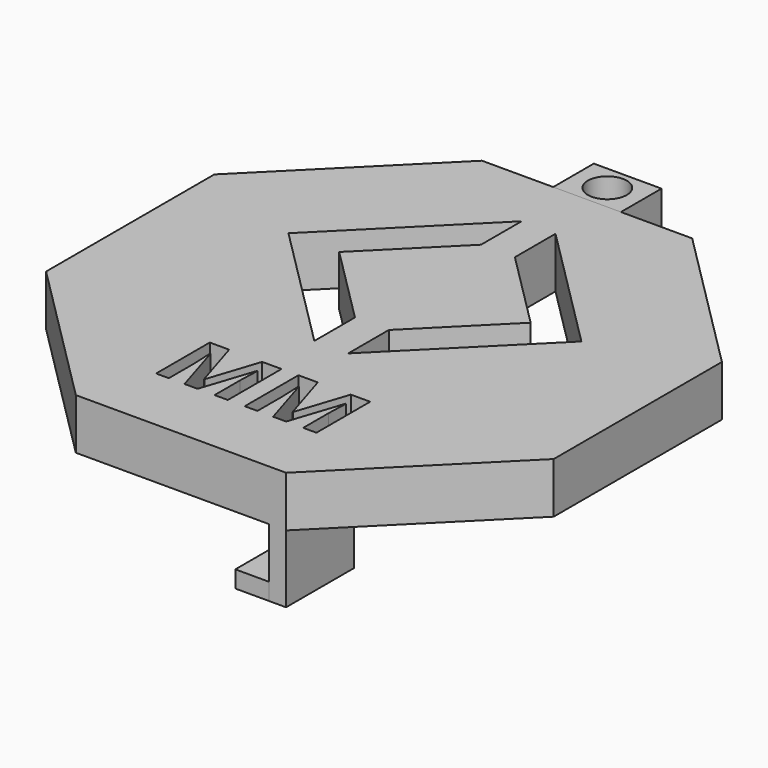
from build123d import *

# Parameters (mm, degrees)
F1_DEPTH     = 3
F2_TEXT_SIZE = 5.5555555556
F3_DEPTH     = 3.001
F4_W         = 1
F4_H         = 5
F5_DEPTH     = 4
F6_W         = 5
F6_H         = 1
F7_DEPTH     = 2
F8_W         = 4
F8_H         = 3
F9_DEPTH     = 3
F10_R        = 1.15
F11_DEPTH    = 3.0010001


# Not quite as in the source:
# - Text() gives the source's letters only with a copy of the font that has no kerning and outlines rounded to 1/6400 em; it was checked with that copy


with BuildPart() as f1:
    # F0 (on Top) → F1 (new body)
    with BuildSketch(Plane.XY):
        Polygon((15, -6.2132034356), (15, 6.2132034356), (6.2132034356, 15), (-6.2132034356, 15), (-15, 6.2132034356), (-15, -6.2132034356), (-6.2132034356, -15), (6.2132034356, -15), align=None)
    extrude(amount=F1_DEPTH)

    # F2 (on face) → F3 (cut, through all)
    with BuildSketch(Plane.XY.offset(3)):
        Polygon((1, 8.418436326), (5.6568542495, 3.7615820765), (1, -0.8952721729), (1, -3.8952721729), (8.6568542495, 3.7615820765), (1, 11.418436326), align=None)
        Polygon((-1, -0.8952721729), (-5.6568542495, 3.7615820765), (-1, 8.418436326), (-1, 11.418436326), (-8.6568542495, 3.7615820765), (-1, -3.8952721729), align=None)
        with Locations((-5.1684027778, -11)):
            Text('MM', F2_TEXT_SIZE, font='Open Sans', font_style=FontStyle.BOLD, text_align=(TextAlign.LEFT, TextAlign.BOTTOM))
    extrude(amount=-F3_DEPTH, mode=Mode.SUBTRACT)

    # F4 (on face) → F5 (join)
    with BuildSketch(Plane(origin=(0, 0, 0), x_dir=(1, 0, 0), z_dir=(0, 0, -1))):
        with Locations((5.7132034356, 12.5)):
            Rectangle(F4_W, F4_H)
    extrude(amount=F5_DEPTH)


with BuildPart() as f7:
    # F6 (on face) → F7 (new body)
    with BuildSketch(Plane(origin=(5.2132034356, 0, 0), x_dir=(0, -1, 0), z_dir=(-1, 0, 0))):
        with Locations((12.5, -3.5)):
            Rectangle(F6_W, F6_H)
    extrude(amount=F7_DEPTH)


with BuildPart() as f9:
    # F8 (on face) → F9 (new body)
    with BuildSketch(Plane(origin=(0, 15, 0), x_dir=(-1, 0, 0), z_dir=(0, 1, 0))):
        with Locations((0, 1.5)):
            Rectangle(F8_W, F8_H)
    extrude(amount=F9_DEPTH)

    # F10 (on face) → F11 (cut, through all)
    with BuildSketch(Plane(origin=(0, 0, 0), x_dir=(1, 0, 0), z_dir=(0, 0, -1))):
        with Locations((0, -16.5)):
            Circle(F10_R)
    extrude(amount=-F11_DEPTH, mode=Mode.SUBTRACT)


solid = Compound([f1.part, f7.part, f9.part])
